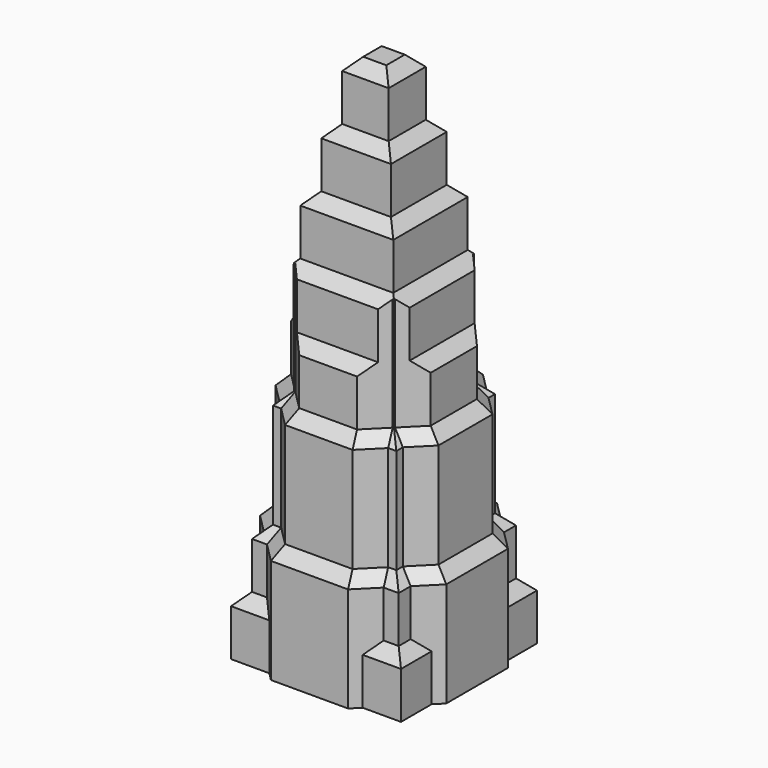
from build123d import *

# Parameters (mm, degrees)
F1_DEPTH     = 25.4
F2_SIZE      = 5.08
F3_DEPTH     = 25.4
F4_SIZE      = 5.08
F5_DEPTH     = 25.4
F6_DEPTH     = 25.4
F7_SIZE      = 5.08
F8_DEPTH     = 25.4
F9_SIZE      = 5.08
F10_DEPTH    = 25.4
F11_T1_DEPTH = 61.5024806542
F11_T3_DEPTH = 61.5024806542
F12_DEPTH    = 25.4
F13_SIZE     = 5.08
F14_DEPTH    = 25.4
F15_SIZE     = 5.08
F16_DEPTH    = 25.4
F17_SIZE     = 5.08


# Not quite as in the source:
# - a fillet or chamfer that OpenCascade refuses, or shapes differently, is made with other operations: its cross-section is extruded or revolved along the edge and cut away or added


with BuildPart() as f1:
    # F0 (on Top) → F1 (new body)
    with BuildSketch(Plane.XY):
        Polygon((37.0489656925, 20.3627443159), (37.0489656925, 37.0489656925), (20.3627443159, 37.0489656925), align=None)
        Polygon((40.5962094665, 16.8155005419), (37.0489656925, 20.3627443159), (37.0489656925, -20.3627443159), (40.5962094665, -16.8155005419), align=None)
        Polygon((37.0489656925, -20.3627443159), (37.0489656925, 20.3627443159), (20.3627443159, 37.0489656925), (-20.3627443159, 37.0489656925), (-37.0489656925, 20.3627443159), (-37.0489656925, -20.3627443159), (-20.3627443159, -37.0489656925), (20.3627443159, -37.0489656925), align=None)
        Polygon((-20.3627443159, 37.0489656925), (20.3627443159, 37.0489656925), (16.8155005419, 40.5962094665), (-16.8155005419, 40.5962094665), align=None)
        Polygon((37.0489656925, -37.0489656925), (37.0489656925, -20.3627443159), (20.3627443159, -37.0489656925), align=None)
        Polygon((-37.0489656925, 20.3627443159), (-20.3627443159, 37.0489656925), (-37.0489656925, 37.0489656925), align=None)
        Polygon((16.8155005419, -40.5962094665), (20.3627443159, -37.0489656925), (-20.3627443159, -37.0489656925), (-16.8155005419, -40.5962094665), align=None)
        Polygon((-37.0489656925, -20.3627443159), (-37.0489656925, 20.3627443159), (-40.5962094665, 16.8155005419), (-40.5962094665, -16.8155005419), align=None)
        Polygon((-37.0489656925, -37.0489656925), (-20.3627443159, -37.0489656925), (-37.0489656925, -20.3627443159), align=None)
    extrude(amount=F1_DEPTH)

    # F2
    f2_edges = [f1.edges().sort_by_distance(p)[0] for p in [
        (-28.705855, 37.048966, 25.4),
        (-37.048966, 28.705855, 25.4),
        (28.705855, 37.048966, 25.4),
        (37.048966, 28.705855, 25.4),
        (37.048966, -28.705855, 25.4),
        (28.705855, -37.048966, 25.4),
        (-28.705855, -37.048966, 25.4),
        (-37.048966, -28.705855, 25.4),
    ]]
    chamfer(f2_edges, length=F2_SIZE)

    # F3 (add): a face of the model
    f3_faces = [f1.faces().sort_by_distance(p)[0] for p in [
        (0, 0, 25.4),
    ]]
    extrude(f3_faces, amount=F3_DEPTH)

    # F4
    f4_edges = [f1.edges().sort_by_distance(p)[0] for p in [
        (-21.129122, 36.282588, 50.8),
        (-28.705855, 31.968966, 50.8),
        (-31.968966, 28.705855, 50.8),
        (-36.282588, 21.129122, 50.8),
        (-40.596209, 0, 50.8),
        (-36.282588, -21.129122, 50.8),
        (-31.968966, -28.705855, 50.8),
        (-28.705855, -31.968966, 50.8),
        (-21.129122, -36.282588, 50.8),
        (0, -40.596209, 50.8),
        (21.129122, -36.282588, 50.8),
        (28.705855, -31.968966, 50.8),
        (31.968966, -28.705855, 50.8),
        (36.282588, -21.129122, 50.8),
        (40.596209, 0, 50.8),
        (36.282588, 21.129122, 50.8),
        (31.968966, 28.705855, 50.8),
        (28.705855, 31.968966, 50.8),
        (21.129122, 36.282588, 50.8),
        (0, 40.596209, 50.8),
    ]]
    chamfer(f4_edges, length=F4_SIZE)

    # F5 (add): a face of the model
    f5_faces = [f1.faces().sort_by_distance(p)[0] for p in [
        (0, 0, 50.8),
    ]]
    extrude(f5_faces, amount=F5_DEPTH)

    # F6 (add): a face of the model
    f6_faces = [f1.faces().sort_by_distance(p)[0] for p in [
        (0, 0, 76.2),
    ]]
    extrude(f6_faces, amount=F6_DEPTH)

    # F7
    f7_edges = [f1.edges().sort_by_distance(p)[0] for p in [
        (-19.024918, 31.202588, 101.6),
        (-25.113753, 26.888966, 101.6),
        (0, 35.516209, 101.6),
        (-26.888966, 25.113753, 101.6),
        (19.024918, 31.202588, 101.6),
        (-31.202588, 19.024918, 101.6),
        (25.113753, 26.888966, 101.6),
        (-35.516209, 0, 101.6),
        (26.888966, 25.113753, 101.6),
        (-31.202588, -19.024918, 101.6),
        (31.202588, 19.024918, 101.6),
        (-26.888966, -25.113753, 101.6),
        (35.516209, 0, 101.6),
        (-25.113753, -26.888966, 101.6),
        (31.202588, -19.024918, 101.6),
        (-19.024918, -31.202588, 101.6),
        (26.888966, -25.113753, 101.6),
        (0, -35.516209, 101.6),
        (25.113753, -26.888966, 101.6),
        (19.024918, -31.202588, 101.6),
    ]]
    chamfer(f7_edges, length=F7_SIZE)

    # F8 (add): a face of the model
    f8_faces = [f1.faces().sort_by_distance(p)[0] for p in [
        (0, 0, 101.6),
    ]]
    extrude(f8_faces, amount=F8_DEPTH)

    # F9
    f9_edges = [f1.edges().sort_by_distance(p)[0] for p in [
        (0, 30.436209, 127),
        (-30.436209, 0, 127),
        (30.436209, 0, 127),
        (0, -30.436209, 127),
    ]]
    chamfer(f9_edges, length=F9_SIZE)

    # F10 (add): a face of the model
    f10_faces = [f1.faces().sort_by_distance(p)[0] for p in [
        (0, 0, 127),
    ]]
    extrude(f10_faces, amount=F10_DEPTH)

    # F11: chamfer of 5.08 on 4 edges, made by hand

    # F11_s2 → F11_t1 (cut)
    with BuildSketch(Plane.XZ.offset(-30.7512403271)):
        Polygon((-25.3562094665, 147.32), (-20.2762094665, 152.4), (-25.3562094665, 152.4), align=None)
        Polygon((25.3562094665, 147.32), (20.2762094665, 152.4), (25.3562094665, 152.4), align=None)
    extrude(amount=F11_T1_DEPTH, mode=Mode.SUBTRACT)

    # F11_s4 → F11_t3 (cut)
    with BuildSketch(Plane.YZ.offset(-30.7512403271)):
        Polygon((-25.3562094665, 147.32), (-20.2762094665, 152.4), (-25.3562094665, 152.4), align=None)
        Polygon((20.2762094665, 152.4), (25.3562094665, 147.32), (25.3562094665, 152.4), align=None)
    extrude(amount=F11_T3_DEPTH, mode=Mode.SUBTRACT)

    # F12 (add): a face of the model
    f12_faces = [f1.faces().sort_by_distance(p)[0] for p in [
        (0, 0, 152.4),
    ]]
    extrude(f12_faces, amount=F12_DEPTH)

    # F13
    f13_edges = [f1.edges().sort_by_distance(p)[0] for p in [
        (0, 20.276209, 177.8),
        (20.276209, 0, 177.8),
        (0, -20.276209, 177.8),
        (-20.276209, 0, 177.8),
    ]]
    chamfer(f13_edges, length=F13_SIZE)

    # F14 (add): a face of the model
    f14_faces = [f1.faces().sort_by_distance(p)[0] for p in [
        (0, 0, 177.8),
    ]]
    extrude(f14_faces, amount=F14_DEPTH)

    # F15
    f15_edges = [f1.edges().sort_by_distance(p)[0] for p in [
        (0, 15.196209, 203.2),
        (-15.196209, 0, 203.2),
        (15.196209, 0, 203.2),
        (0, -15.196209, 203.2),
    ]]
    chamfer(f15_edges, length=F15_SIZE)

    # F16 (add): a face of the model
    f16_faces = [f1.faces().sort_by_distance(p)[0] for p in [
        (0, 0, 203.2),
    ]]
    extrude(f16_faces, amount=F16_DEPTH)

    # F17
    f17_edges = [f1.edges().sort_by_distance(p)[0] for p in [
        (0, 10.116209, 228.6),
        (-10.116209, 0, 228.6),
        (10.116209, 0, 228.6),
        (0, -10.116209, 228.6),
    ]]
    chamfer(f17_edges, length=F17_SIZE)


solid = f1.part
